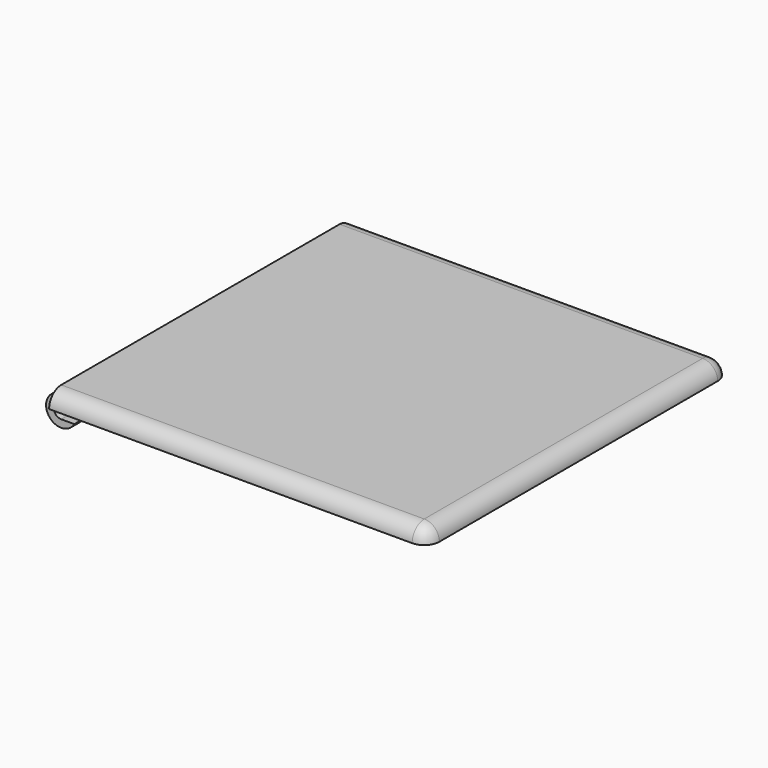
from build123d import *

# Parameters (mm, degrees)
F0_W         = 50
F0_H         = 50
F1_DEPTH     = 2
F2_W         = 2
F2_H         = 1
F3_DEPTH     = 25
F5_DEPTH     = 46
F6_DEPTH     = 25
F8_DEPTH     = 46
F10_DEPTH    = 46
F11_T1_DEPTH = 52.3397459622
F12_R        = 1.99999
F13_T1_DEPTH = 7
F13_T4_ANGLE = 90
F13_T6_ANGLE = 90


# Not quite as in the source:
# - a fillet or chamfer that OpenCascade refuses, or shapes differently, is made with other operations: its cross-section is extruded or revolved along the edge and cut away or added
# - a fillet or chamfer is up to 0.001 mm smaller than in the source, because OpenCascade refuses the exact size


with BuildPart() as f1:
    # F0 (on Top) → F1 (new body)
    with BuildSketch(Plane.XY):
        with Locations((10.2837480605, 1.0400783271)):
            Rectangle(F0_W, F0_H)
    extrude(amount=F1_DEPTH)

    # F12 (radius 2 in the source; OpenCascade refuses exactly that, so slightly less here)
    f12_edges = [f1.edges().sort_by_distance(p)[0] for p in [
        (10.283748, -23.959922, 2),
        (35.283748, 1.040078, 2),
        (10.283748, 26.040078, 2),
    ]]
    fillet(f12_edges, radius=F12_R)

    # F13: fillet of radius 2 on 4 edges, made by hand

    # F13_s2 → F13_t1 (cut)
    with BuildSketch(Plane.XY.offset(-5)):
        with BuildLine():
            ThreePointArc((33.2837480605, -23.9599216729), (34.6979616228, -23.3741352353), (35.2837480605, -21.9599216729))
            Line((35.2837480605, -21.9599216729), (35.2837480605, -23.9599216729))
            Line((35.2837480605, -23.9599216729), (33.2837480605, -23.9599216729))
        make_face()
        with BuildLine():
            ThreePointArc((35.2837480605, 24.0400783271), (34.6979616228, 25.4542918894), (33.2837480605, 26.0400783271))
            Line((33.2837480605, 26.0400783271), (35.2837480605, 26.0400783271))
            Line((35.2837480605, 26.0400783271), (35.2837480605, 24.0400783271))
        make_face()
    extrude(amount=F13_T1_DEPTH, mode=Mode.SUBTRACT)

    # F13_s3 → F13_t4 (revolve, cut)
    with BuildSketch(Plane.YZ.offset(33.2837480605)):
        with BuildLine():
            ThreePointArc((-21.9599316729, 2), (-23.3741381642, 1.4142164913), (-23.9599216729, 1e-05))
            Line((-23.9599216729, 1e-05), (-23.9599216729, 2))
            Line((-23.9599216729, 2), (-21.9599316729, 2))
        make_face()
    revolve(axis=Axis((33.2837480605, -21.9599216729, 2), (0, 0, 1)), revolution_arc=F13_T4_ANGLE, mode=Mode.SUBTRACT)

    # F13_s5 → F13_t6 (revolve, cut)
    with BuildSketch(Plane.XZ.offset(-24.0400783271)):
        with BuildLine():
            ThreePointArc((33.2837580605, 2), (34.6979645518, 1.4142164913), (35.2837480605, 1e-05))
            Line((35.2837480605, 1e-05), (35.2837480605, 2))
            Line((35.2837480605, 2), (33.2837580605, 2))
        make_face()
    revolve(axis=Axis((33.2837480605, 24.0400783271, 2), (0, 0, 1)), revolution_arc=F13_T6_ANGLE, mode=Mode.SUBTRACT)


with BuildPart() as f3:
    # F2 (on face) → F3 (new body)
    with BuildSketch(Plane(origin=(-14.7162519395, 0, 0), x_dir=(0, -1, 0), z_dir=(-1, 0, 0))):
        with Locations((22.9599216729, -0.5)):
            Rectangle(F2_W, F2_H)
    extrude(amount=-F3_DEPTH)

    # F6 (cut): a face of the model
    f6_faces = [f3.faces().sort_by_distance(p)[0] for p in [
        (-14.7162519395, -22.9599216729, -0.5),
    ]]
    extrude(f6_faces, amount=-F6_DEPTH, mode=Mode.SUBTRACT)


with BuildPart() as f5:
    # F4 (on face) → F5 (new body)
    with BuildSketch(Plane(origin=(0, -21.9599216729, 0), x_dir=(-1, 0, 0), z_dir=(0, 1, 0))):
        with BuildLine():
            ThreePointArc((14.7162519395, 0), (15.4233587207, -0.2928932188), (15.7162519395, -1))
            ThreePointArc((15.7162519395, -1), (14.7162519395, -2), (13.7162519395, -1))
            Line((13.7162519395, -1), (12.7162519395, -1))
            ThreePointArc((12.7162519395, -1), (14.7162519395, -3), (16.7162519395, -1))
            ThreePointArc((16.7162519395, -1), (15.2338900297, 0.9318516526), (12.984201132, 0))
            Line((12.984201132, 0), (14.7162519395, 0))
        make_face()
        with BuildLine():
            ThreePointArc((13.7162519395, -1), (14.0091451583, -0.2928932188), (14.7162519395, 0))
            Line((14.7162519395, 0), (12.984201132, 0))
            ThreePointArc((12.984201132, 0), (12.784400287, -0.4823619098), (12.7162519395, -1))
            Line((12.7162519395, -1), (13.7162519395, -1))
        make_face()
    extrude(amount=F5_DEPTH)

    # F7 (on face) → F8 (cut)
    with BuildSketch(Plane.XZ.offset(21.9599216729)):
        with BuildLine():
            ThreePointArc((-13.7162519395, -1), (-14.0091451583, -1.7071067812), (-14.7162519395, -2))
            Line((-14.7162519395, -2), (-12.984201132, -2))
            ThreePointArc((-12.984201132, -2), (-12.784400287, -1.5176380902), (-12.7162519395, -1))
            ThreePointArc((-12.7162519395, -1), (-12.784400287, -0.4823619098), (-12.984201132, 0))
            Line((-12.984201132, 0), (-14.7162519395, 0))
            ThreePointArc((-14.7162519395, 0), (-14.0091451583, -0.2928932188), (-13.7162519395, -1))
        make_face()
    extrude(amount=-F8_DEPTH, mode=Mode.SUBTRACT)

    # F9 (on face) → F10 (join)
    with BuildSketch(Plane.XZ.offset(21.9599216729)):
        with BuildLine():
            ThreePointArc((-15.7162519395, 0.7320508076), (-15.2338900297, 0.9318516526), (-14.7162519395, 1))
            Line((-14.7162519395, 1), (-14.7162519395, 2))
            Line((-14.7162519395, 2), (-15.7162519395, 2))
            Line((-15.7162519395, 2), (-15.7162519395, 0.7320508076))
        make_face()
    extrude(amount=-F10_DEPTH)

    # F11: fillet of radius 5 on 1 edges, made by hand

    # F11_s2 → F11_t1 (cut)
    with BuildSketch(Plane.XZ.offset(-27.2099513081)):
        with BuildLine():
            add(Edge.make_bspline(
                [(-14.7162519395, 2), (-15.319989957, 1.4478409987), (-15.7162519395, 0.7320508076)],
                knots=[0, 0, 0, 1, 1, 1], degree=2, weights=[1, 1, 1]))
            Line((-15.7162519395, 0.7320508076), (-15.8037401736, 0.780484359))
            ThreePointArc((-15.8037401736, 0.780484359), (-15.8162519395, 1.3660254038), (-15.8162519395, 2))
            Line((-15.8162519395, 2), (-15.7162519395, 2.1))
            ThreePointArc((-15.7162519395, 2.1), (-15.2162519395, 2.1), (-14.7837401736, 2.0737925353))
            Line((-14.7837401736, 2.0737925353), (-14.7162519395, 2))
        make_face()
    extrude(amount=F11_T1_DEPTH, mode=Mode.SUBTRACT)


solid = Compound([f1.part, f5.part])
